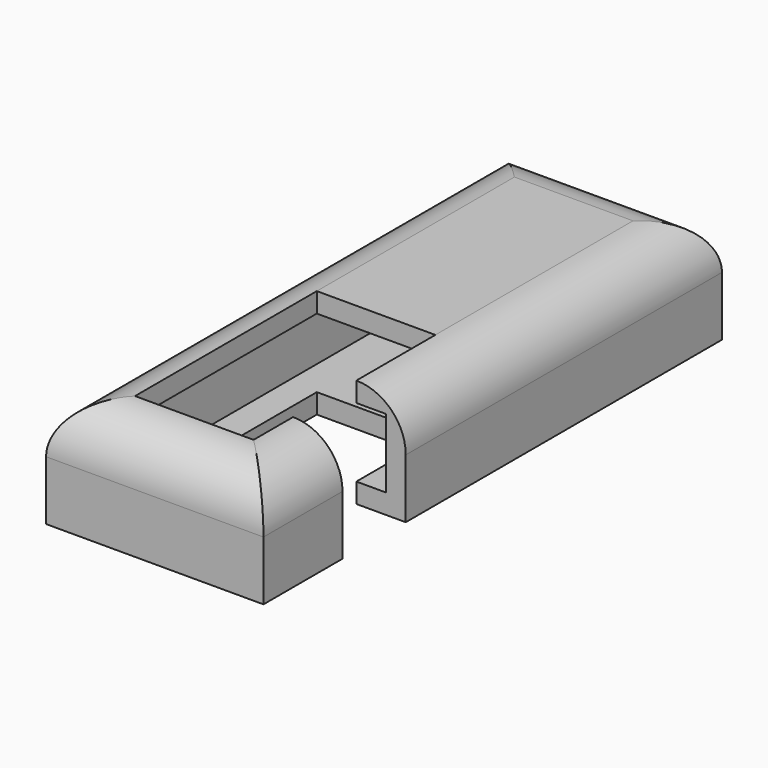
from build123d import *

# Parameters (mm, degrees)
F1_DEPTH    = 11
F2_T        = -2
F3_DEPTH    = 25
F4_DEPTH    = 2
F5_DEPTH    = 2
F6_DEPTH    = 1
F7_T1_DEPTH = 65
F7_T3_DEPTH = 47
F7_T5_DEPTH = 83
F7_T7_DEPTH = 35


# Not quite as in the source:
# - a fillet or chamfer that OpenCascade refuses, or shapes differently, is made with other operations: its cross-section is extruded or revolved along the edge and cut away or added


with BuildPart() as f1:
    # F0 (on Top) → F1 (new body)
    with BuildSketch(Plane.XY):
        Polygon((11, -15), (11, 25), (-11, 25), (-11, -33), (11, -33), (11, -23), (6, -23), (6, -28), (-6, -28), (-6, -15), (-6, -5), (6, -5), (6, -15), align=None)
    extrude(amount=-F1_DEPTH)

    # F2
    f2_openings = [f1.faces().sort_by_distance(p)[0] for p in [
        (0, 25, -5.5),
    ]]
    offset(amount=F2_T, openings=f2_openings, kind=Kind.INTERSECTION)

    # F3 (cut): a face of the model
    f3_faces = [f1.faces().sort_by_distance(p)[0] for p in [
        (0, -3, -5.5),
    ]]
    extrude(f3_faces, amount=-F3_DEPTH, mode=Mode.SUBTRACT)

    # F4 (add): a face of the model
    f4_faces = [f1.faces().sort_by_distance(p)[0] for p in [
        (8, -14, -5.5),
    ]]
    extrude(f4_faces, amount=-F4_DEPTH)

    # F5 (add): a face of the model
    f5_faces = [f1.faces().sort_by_distance(p)[0] for p in [
        (8, -14, -5.5),
    ]]
    extrude(f5_faces, amount=-F5_DEPTH)

    # F6 (cut): faces of the model
    f6_faces = [f1.faces().sort_by_distance(p)[0] for p in [
        (8, -14, -5.5),
        (8, -24, -5.5),
    ]]
    extrude(f6_faces, amount=-F6_DEPTH, mode=Mode.SUBTRACT)

    # F7: fillet of radius 5 on 5 edges, made by hand

    # F7_s2 → F7_t1 (cut)
    with BuildSketch(Plane.XZ.offset(-37.5)):
        with BuildLine():
            ThreePointArc((11, -5), (9.5355339059, -1.4644660941), (6, 0))
            Line((6, 0), (11, 0))
            Line((11, 0), (11, -5))
        make_face()
    extrude(amount=F7_T1_DEPTH, mode=Mode.SUBTRACT)

    # F7_s4 → F7_t3 (cut)
    with BuildSketch(Plane.YZ.offset(-23.5)):
        with BuildLine():
            ThreePointArc((20, 0), (23.5355339059, -1.4644660941), (25, -5))
            Line((25, -5), (25, 0))
            Line((25, 0), (20, 0))
        make_face()
        with BuildLine():
            ThreePointArc((-33, -5), (-31.5355339059, -1.4644660941), (-28, 0))
            Line((-28, 0), (-33, 0))
            Line((-33, 0), (-33, -5))
        make_face()
    extrude(amount=F7_T3_DEPTH, mode=Mode.SUBTRACT)

    # F7_s6 → F7_t5 (cut)
    with BuildSketch(Plane.XZ.offset(-37.5)):
        with BuildLine():
            ThreePointArc((-11, -5), (-9.5355339059, -1.4644660941), (-6, 0))
            Line((-6, 0), (-11, 0))
            Line((-11, 0), (-11, -5))
        make_face()
    extrude(amount=F7_T5_DEPTH, mode=Mode.SUBTRACT)

    # F7_s8 → F7_t7 (cut)
    with BuildSketch(Plane.XZ.offset(10.5)):
        with BuildLine():
            ThreePointArc((11, -5), (9.5355339059, -1.4644660941), (6, 0))
            Line((6, 0), (11, 0))
            Line((11, 0), (11, -5))
        make_face()
    extrude(amount=F7_T7_DEPTH, mode=Mode.SUBTRACT)


solid = f1.part
